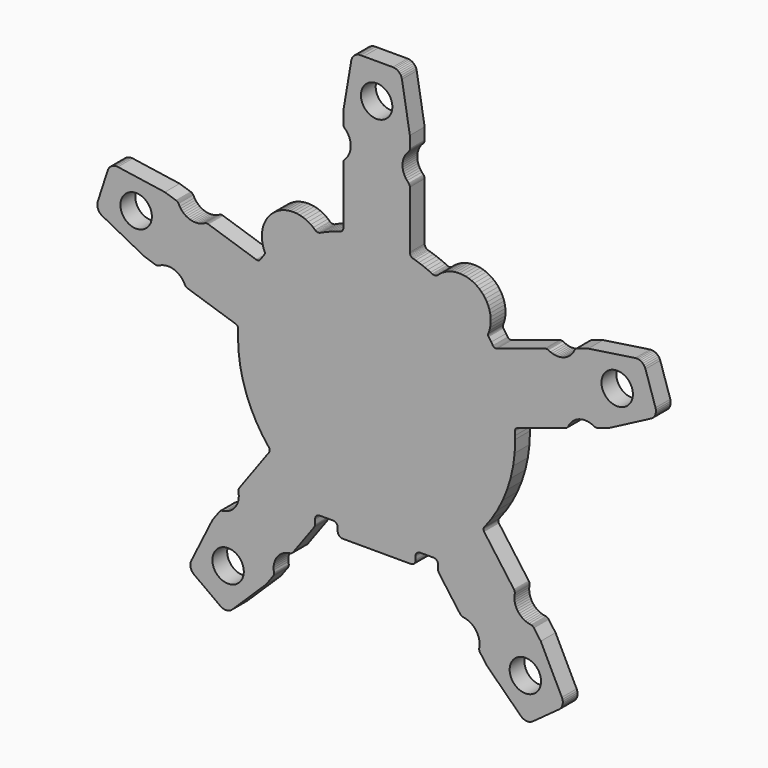
from build123d import *

# Parameters (mm, degrees)
F1_R     = 1.7
F2_DEPTH = 2


# Not quite as in the source:
# - ends of sketch curves that miss each other by under 0.0002 mm in the source are joined


with BuildPart() as f2:
    # F1 (on Front) → F2 (new body)
    with BuildSketch(Plane.XZ):
        Polygon((30.20915, 5.07585), (30.23155, 5.24735), (30.22365, 5.42305), (30.18365, 5.59805), (29.09915, 8.93775), (29.02815, 9.10315), (28.93175, 9.24955), (28.81255, 9.37565), (28.67435, 9.47865), (28.52075, 9.55645), (28.35505, 9.60715), (28.18075, 9.62815), (28.00085, 9.61785), (22.91725, 8.86815), (21.71215, 8.47675), (21.66395, 8.45815), (21.61815, 8.43515), (21.57505, 8.40755), (21.53515, 8.37555), (21.49825, 8.33965), (21.46555, 8.30005), (21.43655, 8.25735), (21.31535, 8.02795), (21.20095, 7.85665), (21.07075, 7.69855), (20.92495, 7.55525), (20.76545, 7.42745), (20.59325, 7.31645), (20.40965, 7.22315), (20.21565, 7.14905), (20.01585, 7.09535), (19.81255, 7.06295), (19.60795, 7.05155), (19.40365, 7.06085), (19.20145, 7.09085), (19.00295, 7.14185), (18.80935, 7.21315), (18.57715, 7.32755), (18.52895, 7.34545), (18.47895, 7.35815), (18.42835, 7.36575), (18.37735, 7.36815), (18.32635, 7.36545), (18.27535, 7.35745), (18.22575, 7.34405), (13.02785, 5.65525), (12.99645, 5.65045), (12.96305, 5.64595), (12.92205, 5.64145), (12.87795, 5.63835), (12.83415, 5.63735), (12.79425, 5.64015), (12.76215, 5.64765), (12.72735, 5.66215), (12.69745, 5.67835), (12.67125, 5.69695), (12.64745, 5.71795), (12.62615, 5.74135), (12.60575, 5.76725), (12.58545, 5.79585), (12.40285, 6.06795), (12.10935, 6.48105), (12.09725, 6.50035), (12.08655, 6.51965), (12.07765, 6.53895), (12.07005, 6.55925), (12.06425, 6.57995), (12.05975, 6.60195), (12.05665, 6.62545), (12.05495, 6.64815), (12.05495, 6.66985), (12.05625, 6.69015), (12.05935, 6.71015), (12.06385, 6.72975), (12.06455, 6.73225), (12.08595, 6.77665), (12.20015, 7.08915), (12.28405, 7.41505), (12.33555, 7.75245), (12.35305, 8.10025), (12.33555, 8.44805), (12.28405, 8.78545), (12.20015, 9.11135), (12.08595, 9.42385), (11.94275, 9.72095), (11.77245, 10.00125), (11.57675, 10.26295), (11.35725, 10.50445), (11.11575, 10.72385), (10.85415, 10.91955), (10.57385, 11.08995), (10.27655, 11.23305), (9.96405, 11.34725), (9.63835, 11.43115), (9.30075, 11.48265), (8.95315, 11.50025), (8.60535, 11.48265), (8.26785, 11.43115), (7.94195, 11.34745), (7.62955, 11.23325), (7.33215, 11.09005), (7.05195, 10.91975), (6.79025, 10.72405), (6.63355, 10.58155), (6.55365, 10.51335), (6.46865, 10.46735), (6.37485, 10.43825), (6.27405, 10.42815), (6.17325, 10.43825), (6.07935, 10.46735), (6.01595, 10.50165), (5.84425, 10.58195), (5.52785, 10.72045), (5.20725, 10.85135), (4.88305, 10.97465), (4.55515, 11.09025), (4.22335, 11.19795), (4.01995, 11.25835), (3.90445, 11.28975), (3.81955, 11.33575), (3.74565, 11.39685), (3.68475, 11.47095), (3.63855, 11.55585), (3.60945, 11.64975), (3.60065, 11.76415), (3.60065, 17.96945), (3.59785, 18.02105), (3.58995, 18.07175), (3.57655, 18.12095), (3.55865, 18.16885), (3.53585, 18.21475), (3.50835, 18.25775), (3.47665, 18.29805), (3.29605, 18.48415), (3.16865, 18.64605), (3.05905, 18.81895), (2.96775, 19.00225), (2.89575, 19.19385), (2.84345, 19.39155), (2.81135, 19.59485), (2.80065, 19.80155), (2.81135, 20.00925), (2.84345, 20.21285), (2.89545, 20.41125), (2.96745, 20.60215), (3.05875, 20.78475), (3.16865, 20.95765), (3.29605, 21.11925), (3.47695, 21.30565), (3.50905, 21.34595), (3.53625, 21.38935), (3.55895, 21.43515), (3.57725, 21.48305), (3.58995, 21.53265), (3.59785, 21.58335), (3.60065, 21.63495), (3.60065, 22.90205), (2.74145, 27.96915), (2.69595, 28.14275), (2.62155, 28.30195), (2.52235, 28.44385), (2.40105, 28.56585), (2.26045, 28.66505), (2.10405, 28.73945), (1.93455, 28.78595), (1.75545, 28.80215), (-1.40005, 28.80225), (-1.70005, 28.80225), (-1.75515, 28.80215), (-1.93425, 28.78595), (-2.10375, 28.73945), (-2.26015, 28.66505), (-2.40075, 28.56585), (-2.52195, 28.44385), (-2.62155, 28.30195), (-2.69565, 28.14275), (-2.74105, 27.96915), (-3.59965, 22.90205), (-3.59965, 21.63495), (-3.59685, 21.58335), (-3.58925, 21.53265), (-3.57615, 21.48305), (-3.55795, 21.43515), (-3.53485, 21.38935), (-3.50765, 21.34595), (-3.47595, 21.30565), (-3.29505, 21.11925), (-3.16755, 20.95765), (-3.05765, 20.78475), (-2.96635, 20.60185), (-2.89405, 20.41065), (-2.84165, 20.21255), (-2.80995, 20.00895), (-2.79895, 19.80155), (-2.80995, 19.59485), (-2.84165, 19.39155), (-2.89405, 19.19385), (-2.96635, 19.00225), (-3.05765, 18.81895), (-3.16755, 18.64605), (-3.29505, 18.48415), (-3.47595, 18.29805), (-3.50765, 18.25775), (-3.53485, 18.21475), (-3.55795, 18.16885), (-3.57615, 18.12095), (-3.58925, 18.07175), (-3.59685, 18.02105), (-3.59965, 17.96945), (-3.59965, 11.83265), (-3.60205, 11.65525), (-3.63115, 11.56135), (-3.67715, 11.47645), (-3.73825, 11.40235), (-3.81235, 11.34125), (-3.89725, 11.29525), (-3.94445, 11.28055), (-3.94495, 11.28045), (-3.99405, 11.26575), (-4.22245, 11.19795), (-4.55425, 11.09025), (-4.88235, 10.97465), (-5.20675, 10.85135), (-5.52735, 10.72045), (-5.84395, 10.58195), (-6.11905, 10.45345), (-6.11985, 10.45415), (-6.21805, 10.42275), (-6.31885, 10.41255), (-6.41955, 10.42275), (-6.51345, 10.45185), (-6.59835, 10.49785), (-6.66105, 10.54975), (-6.66175, 10.54935), (-6.85385, 10.72385), (-7.11545, 10.91955), (-7.39575, 11.08995), (-7.69305, 11.23305), (-8.00555, 11.34725), (-8.33125, 11.43115), (-8.66885, 11.48265), (-9.01655, 11.50025), (-9.36415, 11.48265), (-9.70175, 11.43115), (-10.02745, 11.34725), (-10.33995, 11.23305), (-10.63725, 11.08995), (-10.91755, 10.91955), (-11.17915, 10.72385), (-11.42065, 10.50445), (-11.64015, 10.26295), (-11.83595, 10.00125), (-12.00635, 9.72095), (-12.14945, 9.42385), (-12.26385, 9.11135), (-12.34755, 8.78545), (-12.39905, 8.44805), (-12.41665, 8.10025), (-12.39905, 7.75245), (-12.34755, 7.41505), (-12.26385, 7.08915), (-12.14945, 6.77665), (-12.09905, 6.67175), (-12.09765, 6.66645), (-12.09315, 6.63955), (-12.09105, 6.61125), (-12.09215, 6.58135), (-12.09525, 6.55715), (-12.09935, 6.53375), (-12.10555, 6.51175), (-12.11345, 6.49035), (-12.12275, 6.47005), (-12.13375, 6.44975), (-12.14625, 6.42935), (-12.44455, 6.00525), (-12.56065, 5.83235), (-12.58445, 5.79855), (-12.60785, 5.76755), (-12.63265, 5.73965), (-12.65955, 5.71455), (-12.68985, 5.69215), (-12.72425, 5.67215), (-12.76455, 5.65525), (-12.79735, 5.64765), (-12.83795, 5.64425), (-12.88205, 5.64425), (-12.92685, 5.64635), (-13.00195, 5.65315), (-13.03365, 5.65735), (-18.22545, 7.34405), (-18.27535, 7.35745), (-18.32605, 7.36545), (-18.37705, 7.36815), (-18.42835, 7.36575), (-18.47895, 7.35815), (-18.52855, 7.34545), (-18.57685, 7.32755), (-18.80905, 7.21345), (-19.00225, 7.14215), (-19.20105, 7.09155), (-19.40325, 7.06155), (-19.60755, 7.05225), (-19.81225, 7.06365), (-20.01545, 7.09605), (-20.21535, 7.14975), (-20.40965, 7.22415), (-20.59355, 7.31715), (-20.76545, 7.42815), (-20.92495, 7.55555), (-21.07035, 7.69855), (-21.20125, 7.85635), (-21.31535, 8.02755), (-21.43655, 8.25735), (-21.46515, 8.30005), (-21.49825, 8.33965), (-21.53475, 8.37555), (-21.57475, 8.40755), (-21.61815, 8.43515), (-21.66365, 8.45815), (-21.71185, 8.47675), (-22.91695, 8.86815), (-28.00125, 9.61715), (-28.18075, 9.62745), (-28.35505, 9.60605), (-28.52075, 9.55545), (-28.67405, 9.47755), (-28.81215, 9.37495), (-28.93105, 9.24885), (-29.02785, 9.10245), (-29.09815, 8.93705), (-30.18335, 5.59805), (-30.22335, 5.42305), (-30.23155, 5.24735), (-30.20885, 5.07585), (-30.15785, 4.91115), (-30.07935, 4.75785), (-29.97525, 4.61965), (-29.84675, 4.49975), (-29.69555, 4.40265), (-25.14175, 2.02065), (-23.93665, 1.62935), (-23.88705, 1.61585), (-23.83605, 1.60795), (-23.78515, 1.60485), (-23.73375, 1.60725), (-23.68315, 1.61485), (-23.63355, 1.62725), (-23.58525, 1.64515), (-23.35245, 1.75955), (-23.15875, 1.83085), (-22.96035, 1.88185), (-22.75845, 1.91215), (-22.55415, 1.92185), (-22.34985, 1.91015), (-22.14625, 1.87735), (-21.94545, 1.82365), (-21.75215, 1.74955), (-21.56855, 1.65615), (-21.39625, 1.54525), (-21.23675, 1.41775), (-21.09105, 1.27445), (-20.96015, 1.11665), (-20.84575, 0.94545), (-20.72445, 0.71605), (-20.69625, 0.67335), (-20.66355, 0.63405), (-20.62695, 0.59825), (-20.58705, 0.56615), (-20.54395, 0.53865), (-20.49845, 0.51515), (-20.45025, 0.49655), (-15.31775, -1.17115), (-15.29195, -1.18015), (-15.25435, -1.19425), (-15.21025, -1.21255), (-15.16275, -1.23495), (-15.11795, -1.26005), (-15.07935, -1.28795), (-15.05215, -1.31765), (-15.03075, -1.35275), (-15.01325, -1.38895), (-15.00015, -1.42575), (-14.98975, -1.46405), (-14.98325, -1.50295), (-14.97945, -1.54255), (-14.97805, -1.58325), (-14.99805, -2.17785), (-14.99945, -2.36355), (-14.94125, -3.69645), (-14.76895, -4.99665), (-14.48815, -6.25925), (-14.10305, -7.47955), (-13.61965, -8.65225), (-13.04225, -9.77255), (-12.37635, -10.83605), (-11.60875, -11.86065), (-11.59565, -11.88305), (-11.58605, -11.90505), (-11.57915, -11.92745), (-11.57435, -11.95055), (-11.57155, -11.97535), (-11.56945, -12.00185), (-11.56845, -12.03115), (-11.57125, -12.06355), (-11.58015, -12.10145), (-11.59325, -12.14175), (-11.60875, -12.18175), (-11.62395, -12.21785), (-11.64705, -12.26785), (-11.65075, -12.27505), (-14.86715, -16.70205), (-14.89535, -16.74545), (-14.91845, -16.79095), (-14.93675, -16.83875), (-14.95055, -16.88805), (-14.95875, -16.93875), (-14.96225, -16.98965), (-14.96015, -17.04105), (-14.92365, -17.29735), (-14.91535, -17.50335), (-14.92845, -17.70765), (-14.96225, -17.90955), (-15.01665, -18.10695), (-15.09075, -18.29775), (-15.18445, -18.48105), (-15.29705, -18.65475), (-15.42795, -18.81625), (-15.57335, -18.96235), (-15.73185, -19.09155), (-15.90235, -19.20385), (-16.08365, -19.29825), (-16.27375, -19.37365), (-16.47185, -19.42955), (-16.72785, -19.47395), (-16.77745, -19.48805), (-16.82535, -19.50705), (-16.87085, -19.53075), (-16.91355, -19.55905), (-16.95275, -19.59145), (-16.98935, -19.62795), (-17.02165, -19.66825), (-17.76655, -20.69285), (-20.04995, -25.29685), (-20.11505, -25.46425), (-20.14845, -25.63655), (-20.15195, -25.80985), (-20.12505, -25.97965), (-20.06995, -26.14295), (-19.98725, -26.29485), (-19.87765, -26.43205), (-19.74195, -26.55015), (-16.90185, -28.61445), (-16.74745, -28.70645), (-16.58315, -28.76815), (-16.41295, -28.80015), (-16.24065, -28.80225), (-16.07085, -28.77505), (-15.90685, -28.71855), (-15.75325, -28.63345), (-15.61405, -28.51935), (-11.94155, -24.92475), (-11.19675, -23.90025), (-11.16885, -23.85685), (-11.14545, -23.81095), (-11.12675, -23.76305), (-11.11335, -23.71345), (-11.10475, -23.66315), (-11.10135, -23.61215), (-11.10305, -23.56055), (-11.14025, -23.30355), (-11.14815, -23.09785), (-11.13545, -22.89325), (-11.10165, -22.69165), (-11.04795, -22.49465), (-10.97385, -22.30375), (-10.88015, -22.12045), (-10.76675, -21.94615), (-10.63655, -21.78495), (-10.49115, -21.63915), (-10.33275, -21.51005), (-10.16185, -21.39735), (-9.98025, -21.30295), (-9.78975, -21.22715), (-9.59135, -21.17135), (-9.33605, -21.12695), (-9.28675, -21.11315), (-9.23885, -21.09415), (-9.19375, -21.07045), (-9.15065, -21.04255), (-9.11105, -21.01015), (-9.07455, -20.97395), (-9.04215, -20.93395), (-6.74995, -17.79225), (-6.70105, -17.70365), (-6.67195, -17.60985), (-6.65975, -17.52045), (-6.65975, -17.02485), (-6.65175, -16.90205), (-6.62265, -16.80815), (-6.57655, -16.72325), (-6.51555, -16.64915), (-6.44165, -16.58815), (-6.35675, -16.54205), (-6.26285, -16.51285), (-6.18415, -16.49795), (-4.70425, -16.49795), (-4.70475, -16.50275), (-4.60405, -16.51285), (-4.51015, -16.54205), (-4.42525, -16.58815), (-4.35115, -16.64915), (-4.29005, -16.72325), (-4.24405, -16.80815), (-4.21495, -16.90205), (-4.20975, -17.05205), (-4.20975, -17.36625), (-4.19545, -17.49495), (-4.16635, -17.58875), (-4.12015, -17.67375), (-4.05915, -17.74775), (-3.98525, -17.80895), (-3.90035, -17.85495), (-3.80645, -17.88405), (-3.70555, -17.89425), (3.71075, -17.89785), (3.81135, -17.88575), (3.90515, -17.85665), (3.99015, -17.81065), (4.06415, -17.74955), (4.12535, -17.67545), (4.17135, -17.59055), (4.20045, -17.49665), (4.21045, -17.36625), (4.21045, -16.99835), (4.22055, -16.89755), (4.24965, -16.80365), (4.29585, -16.71875), (4.35685, -16.64465), (4.43075, -16.58365), (4.51565, -16.53755), (4.60955, -16.50845), (4.71035, -16.49825), (4.71045, -16.49795), (6.16005, -16.49795), (6.16005, -16.49825), (6.26075, -16.50845), (6.35465, -16.53755), (6.43955, -16.58365), (6.51365, -16.64465), (6.57475, -16.71875), (6.62075, -16.80365), (6.64985, -16.89755), (6.66005, -16.99835), (6.66045, -16.99835), (6.66045, -17.52165), (6.67335, -17.60925), (6.70245, -17.70315), (6.74855, -17.78805), (6.76415, -17.80705), (9.04045, -20.92985), (9.07285, -20.96945), (9.10935, -21.00595), (9.14935, -21.03805), (9.19205, -21.06625), (9.23755, -21.09005), (9.28505, -21.10895), (9.33435, -21.12275), (9.58925, -21.16725), (9.78735, -21.22305), (9.97825, -21.29885), (10.15945, -21.39325), (10.33025, -21.50585), (10.48945, -21.63505), (10.63485, -21.78075), (10.76505, -21.94205), (10.87845, -22.11635), (10.97245, -22.29965), (11.04615, -22.49045), (11.10025, -22.68755), (11.13365, -22.88875), (11.14675, -23.09305), (11.13855, -23.29865), (11.10165, -23.55535), (11.09955, -23.60665), (11.10305, -23.65805), (11.11165, -23.70865), (11.12545, -23.75825), (11.14405, -23.80615), (11.16745, -23.85195), (11.19565, -23.89535), (11.93985, -24.91995), (15.61305, -28.51455), (15.75215, -28.62825), (15.90585, -28.71365), (16.06945, -28.76985), (16.23935, -28.79705), (16.41155, -28.79505), (16.58175, -28.76295), (16.74575, -28.70125), (16.90005, -28.60895), (19.74095, -26.54605), (19.87595, -26.42755), (19.98585, -26.29045), (20.06885, -26.13815), (20.12405, -25.97485), (20.15085, -25.80465), (20.14775, -25.63175), (20.11435, -25.45915), (20.04895, -25.29135), (17.76485, -20.68805), (17.02065, -19.66345), (16.98825, -19.62315), (16.95175, -19.58665), (16.91215, -19.55425), (16.86905, -19.52595), (16.82365, -19.50215), (16.77605, -19.48325), (16.72645, -19.46915), (16.47085, -19.42465), (16.27235, -19.36885), (16.08155, -19.29345), (15.90035, -19.19935), (15.72945, -19.08705), (15.57065, -18.95785), (15.42525, -18.81185), (15.29465, -18.65055), (15.18205, -18.47655), (15.08835, -18.29335), (15.01425, -18.10215), (14.96015, -17.90505), (14.92635, -17.70315), (14.91335, -17.49855), (14.92125, -17.29285), (14.95845, -17.03625), (14.96015, -16.98485), (14.95705, -16.93385), (14.94845, -16.88325), (14.93505, -16.83395), (14.91645, -16.78605), (14.89335, -16.74065), (14.86545, -16.69725), (11.62805, -12.24065), (11.60775, -12.19345), (11.59605, -12.16345), (11.58465, -12.13035), (11.57465, -12.09625), (11.56775, -12.06385), (11.56605, -12.03595), (11.56915, -11.99845), (11.57465, -11.96395), (11.58365, -11.93165), (11.59535, -11.90095), (11.60975, -11.87135), (11.62735, -11.84235), (11.64765, -11.81305), (11.67115, -11.78315), (12.41185, -10.78545), (13.06915, -9.72635), (13.63895, -8.61195), (14.11615, -7.44575), (14.49575, -6.23305), (14.77305, -4.97875), (14.94255, -3.68715), (15.00045, -2.36355), (14.99495, -1.99355), (14.97845, -1.58495), (14.97875, -1.54535), (14.98115, -1.50705), (14.98635, -1.46985), (14.99495, -1.43405), (15.00665, -1.39855), (15.02325, -1.36375), (15.04425, -1.32865), (15.06385, -1.30585), (15.09005, -1.28355), (15.12105, -1.26175), (15.15275, -1.24185), (15.18235, -1.22495), (15.20715, -1.21145), (15.23095, -1.19975), (20.45125, 0.49655), (20.49915, 0.51515), (20.54465, 0.53865), (20.58775, 0.56655), (20.62765, 0.59855), (20.66415, 0.63435), (20.69695, 0.67405), (20.72555, 0.71635), (20.84615, 0.94515), (20.96045, 1.11635), (21.09135, 1.27415), (21.23745, 1.41745), (21.39735, 1.54525), (21.56955, 1.65615), (21.75285, 1.74955), (21.94645, 1.82365), (22.14735, 1.87735), (22.35055, 1.91015), (22.55485, 1.92185), (22.75885, 1.91215), (22.96075, 1.88185), (23.15915, 1.83085), (23.35205, 1.75955), (23.58525, 1.64515), (23.63385, 1.62725), (23.68345, 1.61485), (23.73415, 1.60725), (23.78545, 1.60485), (23.83645, 1.60795), (23.88705, 1.61585), (23.93705, 1.62935), (25.14215, 2.02065), (29.69515, 4.40335), (29.84675, 4.50045), (29.97525, 4.62005), (30.07965, 4.75815), (30.15815, 4.91145), align=None)
        with Locations((-16.07245, -24.51495)):
            Circle(F1_R, mode=Mode.SUBTRACT)
        with Locations((16.09975, -24.50145)):
            Circle(F1_R, mode=Mode.SUBTRACT)
        with Locations((-26.02335, 6.07795)):
            Circle(F1_R, mode=Mode.SUBTRACT)
        with Locations((26.03495, 6.08635)):
            Circle(F1_R, mode=Mode.SUBTRACT)
        with Locations((0.00275, 24.99905)):
            Circle(F1_R, mode=Mode.SUBTRACT)
    extrude(amount=F2_DEPTH)


solid = f2.part
